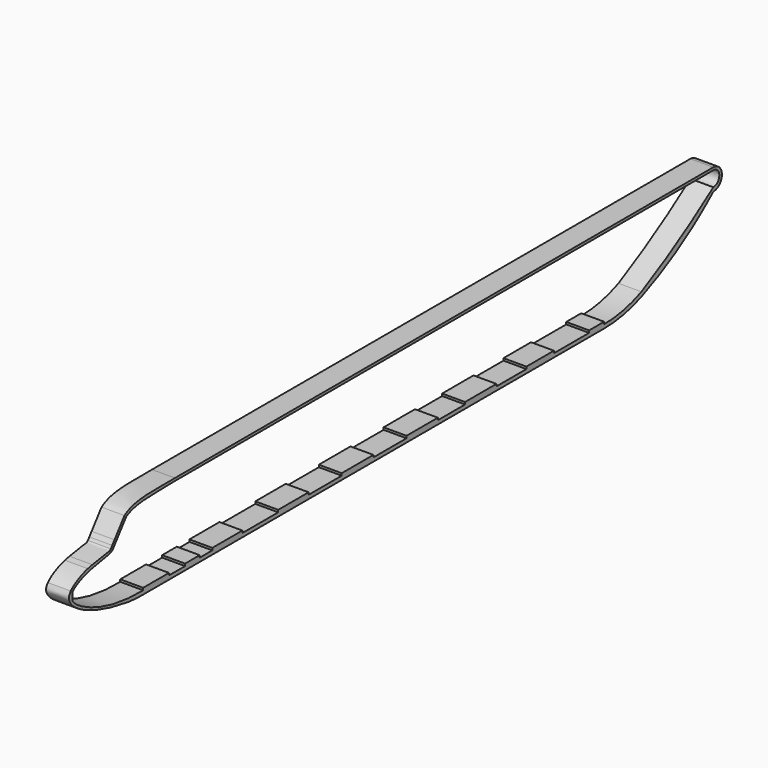
from build123d import *

# Parameters (mm, degrees)
F0_W     = 7.9592205584
F0_H     = 0.9682481177
F0_W_2   = 16.3772823289
F0_W_3   = 16.5999415331
F0_W_4   = 59.5395565033
F0_H_2   = 1.1446848512
F0_W_5   = 17.2708854079
F0_W_6   = 17.1027556062
F0_W_7   = 8.1813335419
F0_W_8   = 17.1027630568
F0_W_9   = 15.0124281645
F1_DEPTH = 10


with BuildPart() as f1:
    # F0 (on Right) → F1 (new body)
    with BuildSketch(Plane.YZ):
        with Locations((-40.2992907912, 1.3097476913)):
            Rectangle(F0_W, F0_H)
        with BuildLine():
            Line((-36.319680512, 0.8256236324), (-44.2789010704, 0.8256236324))
            Line((-44.2789010704, 0.8256236324), (-47.2884887369, 0.8256236324))
            add(Edge.make_bspline(
                [(-47.2884887369, 0.8256236324), (-51.1986791226, -0.4227987286), (-54.7682639191, 0.488674187), (-57.7987805009, 0.8256236324)],
                knots=[0.8788153386, 0.8788153386, 0.8788153386, 0.8788153386, 0.9375977313, 0.9375977313, 0.9375977313, 0.9375977313], degree=3))
            Line((-57.7987805009, 0.8256236324), (-67.1432688832, 0.8256236324))
            add(Edge.make_bspline(
                [(-67.1432688832, 0.8256236324), (-66.6509193776, -0.3373995266), (-66.5816717743, -0.6583984415), (-67.1432688832, -0.8256236324)],
                knots=[0.9569663892, 0.9569663892, 0.9569663892, 0.9569663892, 1, 1, 1, 1], degree=3))
            Line((-67.1432688832, -0.8256236324), (67.1432688832, -0.8256236324))
            Line((67.1432688832, -0.8256236324), (67.1432688832, 0.8256236324))
            Line((67.1432688832, 0.8256236324), (58.3999119699, 0.8256236324))
            Line((58.3999119699, 0.8256236324), (41.129026562, 0.8256236324))
            Line((41.129026562, 0.8256236324), (23.0985023081, 0.8256236324))
            Line((23.0985023081, 0.8256236324), (6.4985607751, 0.8256236324))
            Line((6.4985607751, 0.8256236324), (-13.0418827757, 0.8256236324))
            Line((-13.0418827757, 0.8256236324), (-29.4191651046, 0.8256236324))
            Line((-29.4191651046, 0.8256236324), (-36.319680512, 0.8256236324))
        make_face()
        with BuildLine():
            add(Edge.make_bspline(
                [(-47.2884887369, 0.8256236324), (-51.1986791226, -0.4227987286), (-54.7682639191, 0.488674187), (-57.7987805009, 0.8256236324)],
                knots=[0.8788153386, 0.8788153386, 0.8788153386, 0.8788153386, 0.9375977313, 0.9375977313, 0.9375977313, 0.9375977313], degree=3))
            Line((-47.2884887369, 0.8256236324), (-53.0654229224, 0.8256236324))
            Line((-53.0654229224, 0.8256236324), (-57.7987805009, 0.8256236324))
        make_face()
        with Locations((-21.2305239402, 1.3097476913)):
            Rectangle(F0_W_2, F0_H)
        with BuildLine():
            Line((-57.7987805009, 0.8256236324), (-53.0654229224, 0.8256236324))
            Line((-53.0654229224, 0.8256236324), (-53.0654229224, 1.7938717501))
            Line((-53.0654229224, 1.7938717501), (-67.1432688832, 1.7938717501))
            Line((-67.1432688832, 1.7938717501), (-67.1432688832, 0.8256236324))
            add(Edge.make_bspline(
                [(-57.7987805009, 0.8256236324), (-61.0159191969, 1.1833227475), (-63.6255527419, 0.8935602649), (-67.1432688832, 0.8256236324)],
                knots=[0.9375977313, 0.9375977313, 0.9375977313, 0.9375977313, 1, 1, 1, 1], degree=3))
        make_face()
        with BuildLine():
            Line((-67.1432688832, 0.8256236324), (-57.7987805009, 0.8256236324))
            add(Edge.make_bspline(
                [(-57.7987805009, 0.8256236324), (-61.0159191969, 1.1833227475), (-63.6255527419, 0.8935602649), (-67.1432688832, 0.8256236324)],
                knots=[0.9375977313, 0.9375977313, 0.9375977313, 0.9375977313, 1, 1, 1, 1], degree=3))
        make_face()
        with BuildLine():
            add(Edge.make_bspline(
                [(-67.1432688832, 0.8256236324), (-66.6509193776, -0.3373995266), (-66.5816717743, -0.6583984415), (-67.1432688832, -0.8256236324)],
                knots=[0.9569663892, 0.9569663892, 0.9569663892, 0.9569663892, 1, 1, 1, 1], degree=3))
            Line((-67.1432688832, 0.8256236324), (-67.1432688832, -0.8256236324))
        make_face()
        with BuildLine():
            Line((-67.1432688832, -0.8256236324), (-67.1432688832, 0.8256236324))
            add(Edge.make_bspline(
                [(-67.1432688832, 0.8256236324), (-72.0758134657, 0.7303628282), (-85.4966418977, 1.4113661542), (-101.3533463283, 7.9149516327), (-105.1493369808, 11.5436915404), (-105.7790592313, 12.5425305242)],
                knots=[0, 0, 0, 0, 0.0875005146, 0.1748037653, 0.2115887997, 0.2115887997, 0.2115887997, 0.2115887997], degree=3))
            add(Edge.make_bspline(
                [(-105.7790592313, 12.5425305242), (-105.9744112307, 12.8523896605), (-106.4393049893, 13.8046586359), (-106.4279219113, 14.6656665162), (-106.1115412671, 15.2586876195)],
                knots=[0.2115887997, 0.2115887997, 0.2115887997, 0.2115887997, 0.2230002275, 0.2475165519, 0.2475165519, 0.2475165519, 0.2475165519], degree=3))
            add(Edge.make_bspline(
                [(-106.1115412671, 15.2586876195), (-106.4280364897, 15.7186574339), (-106.5937697782, 16.1640910139), (-106.5921410918, 16.585284844)],
                knots=[0.9836293826, 0.9836293826, 0.9836293826, 0.9836293826, 1, 1, 1, 1], degree=3))
            add(Edge.make_bspline(
                [(-75.376854734, -0.3492794788), (-78.5187930994, 0.100372638), (-90.3610848386, 2.295926245), (-102.7291777595, 7.2472073243), (-108.1012203128, 12.9893553032), (-107.5215165975, 15.5146137824), (-106.5921410918, 16.585284844)],
                knots=[0.0801395338, 0.0801395338, 0.0801395338, 0.0801395338, 0.1438178441, 0.2897928885, 0.3749773752, 0.4363049571, 0.4363049571, 0.4363049571, 0.4363049571], degree=3))
            ThreePointArc((-75.376854734, -0.3492794788), (-71.2669456321, -0.7064381134), (-67.1432688832, -0.8256236324))
        make_face()
        with Locations((14.7985315416, 1.3097476913)):
            Rectangle(F0_W_3, F0_H)
        with BuildLine():
            Line((-49.8266220093, 35.7562787831), (-29.3324157713, 35.7562787831))
            add(Edge.make_bspline(
                [(-31.3463312427, 36.9009636343), (-30.6162211649, 36.6342598411), (-29.9359409959, 36.264957093), (-29.3600573473, 35.7800296462), (-29.3324157713, 35.7562787831)],
                knots=[0.5476252208, 0.5476252208, 0.5476252208, 0.5476252208, 0.5656279815, 0.5665441357, 0.5665441357, 0.5665441357, 0.5665441357], degree=3))
            Line((-31.3463312427, 36.9009636343), (-41.4767201262, 36.9009636343))
            add(Edge.make_bspline(
                [(-49.8266220093, 35.7562787831), (-46.6034582942, 35.95606144), (-43.9288870011, 36.4255610772), (-41.4767201262, 36.9009636343)],
                knots=[0.5976663005, 0.5976663005, 0.5976663005, 0.5976663005, 0.6382752389, 0.6382752389, 0.6382752389, 0.6382752389], degree=3))
        make_face()
        with BuildLine():
            add(Edge.make_bspline(
                [(-31.3463312427, 36.9009636343), (-30.6162211649, 36.6342598411), (-29.9359409959, 36.264957093), (-29.3600573473, 35.7800296462), (-29.3324157713, 35.7562787831)],
                knots=[0.5476252208, 0.5476252208, 0.5476252208, 0.5476252208, 0.5656279815, 0.5665441357, 0.5665441357, 0.5665441357, 0.5665441357], degree=3))
            Line((-29.3324157713, 35.7562787831), (-27.0790393766, 35.7562787831))
            add(Edge.make_bspline(
                [(-27.9329801586, 36.9009636343), (-27.5874335917, 36.590939793), (-27.2981663641, 36.213302791), (-27.0790393766, 35.7562787831)],
                knots=[0.7220869644, 0.7220869644, 0.7220869644, 0.7220869644, 0.7320653179, 0.7320653179, 0.7320653179, 0.7320653179], degree=3))
            Line((-27.9329801586, 36.9009636343), (-31.3463312427, 36.9009636343))
        make_face()
        with BuildLine():
            add(Edge.make_bspline(
                [(-27.9329801586, 36.9009636343), (-27.5874335917, 36.590939793), (-27.2981663641, 36.213302791), (-27.0790393766, 35.7562787831)],
                knots=[0.7220869644, 0.7220869644, 0.7220869644, 0.7220869644, 0.7320653179, 0.7320653179, 0.7320653179, 0.7320653179], degree=3))
            Line((-27.0790393766, 35.7562787831), (184.205442667, 35.7562787831))
            Line((184.205442667, 35.7562787831), (184.205442667, 36.9009636343))
            Line((184.205442667, 36.9009636343), (-27.9329801586, 36.9009636343))
        make_face()
        with BuildLine():
            Line((-83.2053124905, 23.9070430398), (-81.5205250131, 26.1137338048))
            add(Edge.make_bspline(
                [(-81.8276049313, 26.3324605583), (-81.7285806251, 26.2701481945), (-81.6261511228, 26.1970663843), (-81.5205250131, 26.1137338048)],
                knots=[0.7832802469, 0.7832802469, 0.7832802469, 0.7832802469, 0.7877852316, 0.7877852316, 0.7877852316, 0.7877852316], degree=3))
            add(Edge.make_bspline(
                [(-83.2053124905, 23.9070430398), (-82.7734139474, 24.5261063334), (-82.337894388, 25.3786099624), (-81.8276049313, 26.3324605583)],
                knots=[0.4237232055, 0.4237232055, 0.4237232055, 0.4237232055, 0.4446888147, 0.4446888147, 0.4446888147, 0.4446888147], degree=3))
        make_face()
        with BuildLine():
            add(Edge.make_bspline(
                [(-81.8276049313, 26.3324605583), (-81.7285806251, 26.2701481945), (-81.6261511228, 26.1970663843), (-81.5205250131, 26.1137338048)],
                knots=[0.7832802469, 0.7832802469, 0.7832802469, 0.7832802469, 0.7877852316, 0.7877852316, 0.7877852316, 0.7877852316], degree=3))
            Line((-81.5205250131, 26.1137338048), (-76.3889253139, 32.834969461))
            add(Edge.make_bspline(
                [(-81.8276049313, 26.3324605583), (-80.6726743978, 28.4912964173), (-79.1347380919, 31.1692780126), (-76.3889253139, 32.834969461)],
                knots=[0.4446888147, 0.4446888147, 0.4446888147, 0.4446888147, 0.4921399658, 0.4921399658, 0.4921399658, 0.4921399658], degree=3))
        make_face()
        with BuildLine():
            Line((-105.7790592313, 12.5425305242), (-105.7790592313, 14.8325555243))
            add(Edge.make_bspline(
                [(-105.7790592313, 14.8325555243), (-105.9036909626, 14.9757756925), (-106.0146769352, 15.1179124494), (-106.1115412671, 15.2586876195)],
                knots=[0.978619105, 0.978619105, 0.978619105, 0.978619105, 0.9836293826, 0.9836293826, 0.9836293826, 0.9836293826], degree=3))
            add(Edge.make_bspline(
                [(-105.7790592313, 12.5425305242), (-105.9744112307, 12.8523896605), (-106.4393049893, 13.8046586359), (-106.4279219113, 14.6656665162), (-106.1115412671, 15.2586876195)],
                knots=[0.2115887997, 0.2115887997, 0.2115887997, 0.2115887997, 0.2230002275, 0.2475165519, 0.2475165519, 0.2475165519, 0.2475165519], degree=3))
        make_face()
        with BuildLine():
            add(Edge.make_bspline(
                [(-105.7790592313, 14.8325555243), (-105.9036909626, 14.9757756925), (-106.0146769352, 15.1179124494), (-106.1115412671, 15.2586876195)],
                knots=[0.978619105, 0.978619105, 0.978619105, 0.978619105, 0.9836293826, 0.9836293826, 0.9836293826, 0.9836293826], degree=3))
            Line((-105.7790592313, 14.8325555243), (-105.7790592313, 15.7497413456))
            add(Edge.make_bspline(
                [(-106.1115412671, 15.2586876195), (-106.0246124997, 15.4216261385), (-105.9143855758, 15.5849789536), (-105.7790592313, 15.7497413456)],
                knots=[0.2475165519, 0.2475165519, 0.2475165519, 0.2475165519, 0.2542526589, 0.2542526589, 0.2542526589, 0.2542526589], degree=3))
        make_face()
        with BuildLine():
            Line((-49.8266220093, 36.9009636343), (-49.8266220093, 35.7562787831))
            add(Edge.make_bspline(
                [(-49.8266220093, 35.7562787831), (-46.6034582942, 35.95606144), (-43.9288870011, 36.4255610772), (-41.4767201262, 36.9009636343)],
                knots=[0.5976663005, 0.5976663005, 0.5976663005, 0.5976663005, 0.6382752389, 0.6382752389, 0.6382752389, 0.6382752389], degree=3))
            Line((-41.4767201262, 36.9009636343), (-49.8266220093, 36.9009636343))
        make_face()
        with BuildLine():
            add(Edge.make_bspline(
                [(-76.3889253139, 32.834969461), (-70.2825284986, 36.5392908326), (-58.2023310565, 35.23712383), (-49.8266220093, 35.7562787831)],
                knots=[0.4921399658, 0.4921399658, 0.4921399658, 0.4921399658, 0.5976663005, 0.5976663005, 0.5976663005, 0.5976663005], degree=3))
            Line((-49.8266220093, 35.7562787831), (-49.8266220093, 36.9009636343))
            add(Edge.make_bspline(
                [(-77.3271471262, 33.6782447994), (-71.0137479896, 37.9678944533), (-59.9470632222, 36.5232924918), (-49.8266220093, 36.9009636343)],
                knots=[0.3035636496, 0.3035636496, 0.3035636496, 0.3035636496, 0.4445217782, 0.4445217782, 0.4445217782, 0.4445217782], degree=3))
            Line((-77.3271471262, 33.6782447994), (-82.7458889947, 26.570704936))
            add(Edge.make_bspline(
                [(-82.7458889947, 26.570704936), (-82.6409378067, 26.595297775), (-82.3634844697, 26.6047383627), (-82.0375313521, 26.4645595549), (-81.8276049313, 26.3324605583)],
                knots=[0.767285406, 0.767285406, 0.767285406, 0.767285406, 0.7737299116, 0.7832802469, 0.7832802469, 0.7832802469, 0.7832802469], degree=3))
            add(Edge.make_bspline(
                [(-81.8276049313, 26.3324605583), (-80.6726743978, 28.4912964173), (-79.1347380919, 31.1692780126), (-76.3889253139, 32.834969461)],
                knots=[0.4446888147, 0.4446888147, 0.4446888147, 0.4446888147, 0.4921399658, 0.4921399658, 0.4921399658, 0.4921399658], degree=3))
        make_face()
        with Locations((213.9752209187, 36.3286212087)):
            Rectangle(F0_W_4, F0_H_2)
        with BuildLine():
            add(Edge.make_bspline(
                [(-83.2053124905, 23.9070430398), (-82.7734139474, 24.5261063334), (-82.337894388, 25.3786099624), (-81.8276049313, 26.3324605583)],
                knots=[0.4237232055, 0.4237232055, 0.4237232055, 0.4237232055, 0.4446888147, 0.4446888147, 0.4446888147, 0.4446888147], degree=3))
            add(Edge.make_bspline(
                [(-82.7458889947, 26.570704936), (-82.6409378067, 26.595297775), (-82.3634844697, 26.6047383627), (-82.0375313521, 26.4645595549), (-81.8276049313, 26.3324605583)],
                knots=[0.767285406, 0.767285406, 0.767285406, 0.767285406, 0.7737299116, 0.7832802469, 0.7832802469, 0.7832802469, 0.7832802469], degree=3))
            Line((-82.7458889947, 26.570704936), (-84.0048450328, 24.9193843076))
            add(Edge.make_bspline(
                [(-94.8389886697, 21.9150389209), (-91.9546645853, 22.3878238509), (-87.3974074928, 22.4492787894), (-84.977370385, 22.3216318756), (-84.2595160002, 24.3097150361), (-84.0048450328, 24.9193843076)],
                knots=[0.5679522733, 0.5679522733, 0.5679522733, 0.5679522733, 0.6501774444, 0.7059587467, 0.7326988833, 0.7326988833, 0.7326988833, 0.7326988833], degree=3))
            add(Edge.make_bspline(
                [(-97.3343178856, 21.3945470699), (-96.4935969707, 21.584978542), (-95.6568843275, 21.7579506298), (-94.8389886865, 21.9150389176)],
                knots=[0.0865231218, 0.0865231218, 0.0865231218, 0.0865231218, 0.1024560332, 0.1024560332, 0.1024560332, 0.1024560332], degree=3))
            add(Edge.make_bspline(
                [(-106.5921410918, 16.585284844), (-104.9529463621, 18.4736909304), (-101.1774679584, 20.4045249526), (-97.3343178855, 21.3945470692)],
                knots=[0.4363049571, 0.4363049571, 0.4363049571, 0.4363049571, 0.5444720527, 0.5444720527, 0.5444720527, 0.5444720527], degree=3))
            add(Edge.make_bspline(
                [(-106.1115412671, 15.2586876195), (-106.4280364897, 15.7186574339), (-106.5937697782, 16.1640910139), (-106.5921410918, 16.585284844)],
                knots=[0.9836293826, 0.9836293826, 0.9836293826, 0.9836293826, 1, 1, 1, 1], degree=3))
            add(Edge.make_bspline(
                [(-106.1115412671, 15.2586876195), (-106.0246124997, 15.4216261385), (-105.9143855758, 15.5849789536), (-105.7790592313, 15.7497413456)],
                knots=[0.2475165519, 0.2475165519, 0.2475165519, 0.2475165519, 0.2542526589, 0.2542526589, 0.2542526589, 0.2542526589], degree=3))
            add(Edge.make_bspline(
                [(-105.7790592313, 15.7497413456), (-104.5149320358, 17.2888401911), (-97.2837116626, 20.7682618377), (-86.1446484374, 21.7822829697), (-83.9828873041, 22.7925034497), (-83.2053124905, 23.9070430398)],
                knots=[0.2542526589, 0.2542526589, 0.2542526589, 0.2542526589, 0.3171768152, 0.3859774667, 0.4237232055, 0.4237232055, 0.4237232055, 0.4237232055], degree=3))
        make_face()
        Polygon((67.1432688832, 0.8256236324), (67.1432688832, -0.8256236324), (184.205442667, -0.8256236324), (184.205442667, 0.8256236324), (176.0241091251, 0.8256236324), (156.8310111761, 0.8256236324), (141.8185830116, 0.8256236324), (125.4759579897, 0.8256236324), (108.3731949329, 0.8256236324), (93.5508012772, 0.8256236324), (76.448045671, 0.8256236324), align=None)
        with Locations((49.7644692659, 1.3097476913)):
            Rectangle(F0_W_5, F0_H)
        with BuildLine():
            Line((243.7449991703, 36.9009636343), (243.7449991703, 35.7562787831))
            ThreePointArc((243.7449991703, 35.7562787831), (247.0123348758, 32.4889430776), (243.7449991703, 29.2216073722))
            Line((243.7449991703, 29.2216073722), (243.7449991703, 27.5277942419))
            ThreePointArc((243.7449991703, 27.5277942419), (248.4315838665, 32.2143789381), (243.7449991703, 36.9009636343))
        make_face()
        with BuildLine():
            Line((184.205442667, 0.8256236324), (184.205442667, -0.8256236324))
            ThreePointArc((184.205442667, -0.8256236324), (194.5543556633, 0.1635588042), (204.5284956694, 3.0952841043))
            ThreePointArc((204.5284956694, 3.0952841043), (218.592518618, 9.8322781675), (231.8167869207, 18.0968143531))
            ThreePointArc((231.8167869207, 18.0968143531), (237.9094832192, 22.6496646882), (243.7449991703, 27.5277942419))
            Line((243.7449991703, 27.5277942419), (243.7449991703, 29.2216073722))
            ThreePointArc((243.7449991703, 29.2216073722), (224.6014403462, 16.3731386899), (204.5284956694, 5.0313626416))
            ThreePointArc((204.5284956694, 5.0313626416), (194.5822765284, 1.8880807661), (184.205442667, 0.8256236324))
        make_face()
        with BuildLine():
            add(Edge.make_bspline(
                [(-94.8389886697, 21.9150389209), (-91.9546645853, 22.3878238509), (-87.3974074928, 22.4492787894), (-84.977370385, 22.3216318756), (-84.2595160002, 24.3097150361), (-84.0048450328, 24.9193843076)],
                knots=[0.5679522733, 0.5679522733, 0.5679522733, 0.5679522733, 0.6501774444, 0.7059587467, 0.7326988833, 0.7326988833, 0.7326988833, 0.7326988833], degree=3))
            Line((-84.0048450328, 24.9193843076), (-84.7766473889, 23.9070430398))
            add(Edge.make_bspline(
                [(-94.8389886697, 21.9150389209), (-91.0215834223, 22.6482249451), (-86.1091370373, 23.2063937055), (-85.1780004227, 23.3783596749), (-84.7766473889, 23.9070430398)],
                knots=[0.1024560332, 0.1024560332, 0.1024560332, 0.1024560332, 0.1768205078, 0.2096643307, 0.2096643307, 0.2096643307, 0.2096643307], degree=3))
        make_face()
        with Locations((84.9994234741, 1.3097476913)):
            Rectangle(F0_W_6, F0_H)
        with Locations((180.1147758961, 1.3097476913)):
            Rectangle(F0_W_7, F0_H)
        with Locations((116.9245764613, 1.3097476913)):
            Rectangle(F0_W_8, F0_H)
        with Locations((149.3247970939, 1.3097476913)):
            Rectangle(F0_W_9, F0_H)
    extrude(amount=F1_DEPTH)


solid = f1.part
